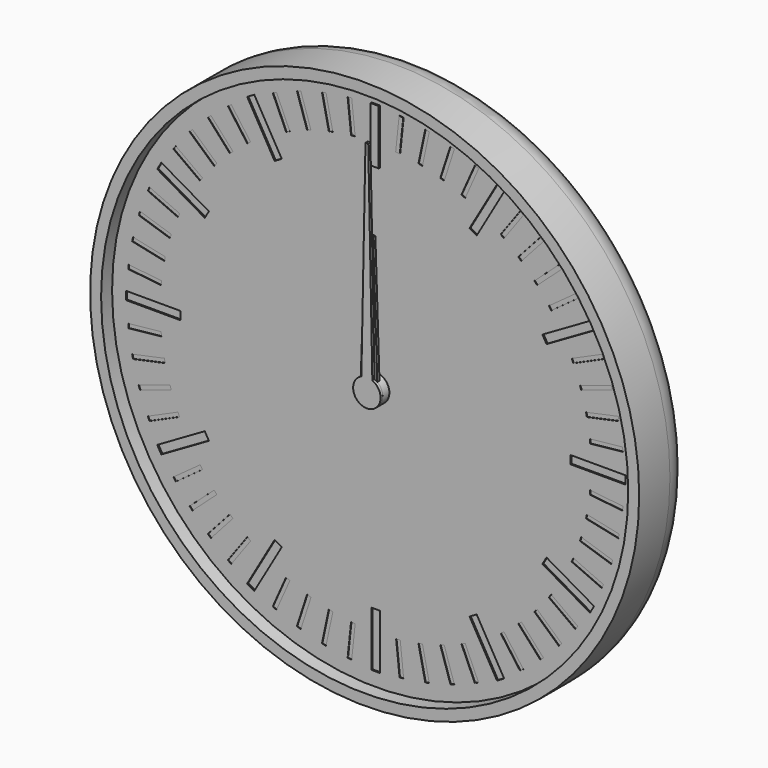
from build123d import *

# Parameters (mm, degrees)
F0_R      = 100
F1_DEPTH  = 24
F2_R      = 10
F3_T      = -4
F4_R      = 5
F4_R_2    = 3
F5_DEPTH  = 2
F6_DEPTH  = 19
F7_DEPTH  = 8
F9_DEPTH  = 4
F11_DEPTH = 4
F12_R     = 5
F12_R_2   = 3
F13_DEPTH = 2
F14_R     = 3
F15_DEPTH = 4
F17_DEPTH = 4
F18_R     = 3
F19_DEPTH = 2
F20_R     = 98
F20_R_2   = 5
F21_DEPTH = 1
F23_R     = 5
F23_R_2   = 3
F24_DEPTH = 2
F25_W     = 3
F25_H     = 20
F25_W_2   = 20
F25_H_2   = 3
F26_DEPTH = 0.5
F27_W     = 1.5
F27_H     = 12
F27_W_2   = 12
F27_H_2   = 1.5
F28_DEPTH = 0.2
F29_DEPTH = 1
F30_DEPTH = 0.4
F31_R     = 5
F31_R_2   = 3
F32_DEPTH = 5
F33_R     = 3
F34_DEPTH = 1
F36_DEPTH = 1


with BuildPart() as f1:
    # F0 (on Front) → F1 (new body)
    with BuildSketch(Plane.XZ):
        Circle(F0_R)
    extrude(amount=F1_DEPTH)

    # F2
    f2_edges = [f1.edges().sort_by_distance(p)[0] for p in [
        (-100, 0, 0),
    ]]
    fillet(f2_edges, radius=F2_R)

    # F3
    f3_openings = [f1.faces().sort_by_distance(p)[0] for p in [
        (0, -24, 0),
    ]]
    offset(amount=F3_T, openings=f3_openings)

    # F4 (on face) → F5 (join)
    with BuildSketch(Plane.XZ.offset(4)):
        Circle(F4_R)
        Circle(F4_R_2, mode=Mode.SUBTRACT)
        with Locations((40, 0)):
            Circle(F4_R)
        with Locations((40, 0)):
            Circle(F4_R_2, mode=Mode.SUBTRACT)
    extrude(amount=F5_DEPTH)


with BuildPart() as f6:
    # F6 (new): a face of the model
    f6_faces = [f1.part.faces().sort_by_distance(p)[0] for p in [
        (0, -4, 0),
    ]]
    extrude(f6_faces, amount=F6_DEPTH)

    # F8 (on face) → F9 (join)
    with BuildSketch(Plane.XZ.offset(6)):
        with BuildLine():
            ThreePointArc((9.2729637667, -1.3794085621), (9.3494561423, -0.6915886375), (9.375, 0))
            ThreePointArc((9.375, 0), (9.3494561423, 0.6915886375), (9.2729637667, 1.3794085621))
            ThreePointArc((9.2729637667, 1.3794085621), (8.9161548403, 2.8970343223), (8.3127812852, 4.3345463782))
            ThreePointArc((8.3127812852, 4.3345463782), (7.5845343223, 5.5104867402), (6.6911892658, 6.566476316))
            ThreePointArc((6.6911892658, 6.566476316), (5.5104867402, 7.5845343223), (4.1773988938, 8.3928519278))
            ThreePointArc((4.1773988938, 8.3928519278), (2.8970343223, 8.9161548403), (1.5536078905, 9.2453733036))
            ThreePointArc((1.5536078905, 9.2453733036), (0, 9.375), (-1.5536078905, 9.2453733036))
            ThreePointArc((-1.5536078905, 9.2453733036), (-2.8970343223, 8.9161548403), (-4.1773988938, 8.3928519278))
            ThreePointArc((-4.1773988938, 8.3928519278), (-5.5104867402, 7.5845343223), (-6.6911892658, 6.566476316))
            ThreePointArc((-6.6911892658, 6.566476316), (-7.5845343223, 5.5104867402), (-8.3127812852, 4.3345463782))
            ThreePointArc((-8.3127812852, 4.3345463782), (-8.9161548403, 2.8970343223), (-9.2729637667, 1.3794085621))
            ThreePointArc((-9.2729637667, 1.3794085621), (-9.375, 0), (-9.2729637667, -1.3794085621))
            ThreePointArc((-9.2729637667, -1.3794085621), (-8.9161548403, -2.8970343223), (-8.3127812852, -4.3345463782))
            ThreePointArc((-8.3127812852, -4.3345463782), (-7.5845343223, -5.5104867402), (-6.6911892658, -6.566476316))
            ThreePointArc((-6.6911892658, -6.566476316), (-5.5104867402, -7.5845343223), (-4.1773988938, -8.3928519278))
            ThreePointArc((-4.1773988938, -8.3928519278), (-2.8970343223, -8.9161548403), (-1.5536078905, -9.2453733036))
            ThreePointArc((-1.5536078905, -9.2453733036), (0, -9.375), (1.5536078905, -9.2453733036))
            ThreePointArc((1.5536078905, -9.2453733036), (2.8970343223, -8.9161548403), (4.1773988938, -8.3928519278))
            ThreePointArc((4.1773988938, -8.3928519278), (5.5104867402, -7.5845343223), (6.6911892658, -6.566476316))
            ThreePointArc((6.6911892658, -6.566476316), (7.5845343223, -5.5104867402), (8.3127812852, -4.3345463782))
            ThreePointArc((8.3127812852, -4.3345463782), (8.9161548403, -2.8970343223), (9.2729637667, -1.3794085621))
        make_face()
        with BuildLine():
            ThreePointArc((8.3127812852, 4.3345463782), (8.9161548403, 2.8970343223), (9.2729637667, 1.3794085621))
            Line((9.2729637667, 1.3794085621), (11.1823199426, 2.3946312492))
            Line((11.1823199426, 2.3946312492), (10.8182678729, 3.515068311))
            Line((10.8182678729, 3.515068311), (10.4542158031, 4.6355053728))
            Line((10.4542158031, 4.6355053728), (8.3127812852, 4.3345463782))
        make_face()
        with BuildLine():
            Line((11.1823199426, -2.3946312492), (9.2729637667, -1.3794085621))
            ThreePointArc((9.2729637667, -1.3794085621), (8.9161548403, -2.8970343223), (8.3127812852, -4.3345463782))
            Line((8.3127812852, -4.3345463782), (10.4542158031, -4.6355053728))
            Line((10.4542158031, -4.6355053728), (10.8182678729, -3.515068311))
            Line((10.8182678729, -3.515068311), (11.1823199426, -2.3946312492))
        make_face()
        with BuildLine():
            ThreePointArc((4.1773988938, 8.3928519278), (5.5104867402, 7.5845343223), (6.6911892658, 6.566476316))
            Line((6.6911892658, 6.566476316), (7.6391579371, 8.5101001246))
            Line((7.6391579371, 8.5101001246), (6.6860572448, 9.202568311))
            Line((6.6860572448, 9.202568311), (5.7329565525, 9.8950364974))
            Line((5.7329565525, 9.8950364974), (4.1773988938, 8.3928519278))
        make_face()
        with BuildLine():
            Line((7.6391579371, -8.5101001246), (6.6911892658, -6.566476316))
            ThreePointArc((6.6911892658, -6.566476316), (5.5104867402, -7.5845343223), (4.1773988938, -8.3928519278))
            Line((4.1773988938, -8.3928519278), (5.7329565525, -9.8950364974))
            Line((5.7329565525, -9.8950364974), (6.6860572448, -9.202568311))
            Line((6.6860572448, -9.202568311), (7.6391579371, -8.5101001246))
        make_face()
        with BuildLine():
            ThreePointArc((-1.5536078905, 9.2453733036), (0, 9.375), (1.5536078905, 9.2453733036))
            Line((1.5536078905, 9.2453733036), (1.1780972451, 11.375))
            Line((1.1780972451, 11.375), (0, 11.375))
            Line((0, 11.375), (-1.1780972451, 11.375))
            Line((-1.1780972451, 11.375), (-1.5536078905, 9.2453733036))
        make_face()
        with BuildLine():
            Line((1.1780972451, -11.375), (1.5536078905, -9.2453733036))
            ThreePointArc((1.5536078905, -9.2453733036), (0, -9.375), (-1.5536078905, -9.2453733036))
            Line((-1.5536078905, -9.2453733036), (-1.1780972451, -11.375))
            Line((-1.1780972451, -11.375), (0, -11.375))
            Line((0, -11.375), (1.1780972451, -11.375))
        make_face()
        with BuildLine():
            ThreePointArc((-6.6911892658, 6.566476316), (-5.5104867402, 7.5845343223), (-4.1773988938, 8.3928519278))
            Line((-4.1773988938, 8.3928519278), (-5.7329565525, 9.8950364974))
            Line((-5.7329565525, 9.8950364974), (-6.6860572448, 9.202568311))
            Line((-6.6860572448, 9.202568311), (-7.6391579371, 8.5101001246))
            Line((-7.6391579371, 8.5101001246), (-6.6911892658, 6.566476316))
        make_face()
        with BuildLine():
            Line((-5.7329565525, -9.8950364974), (-4.1773988938, -8.3928519278))
            ThreePointArc((-4.1773988938, -8.3928519278), (-5.5104867402, -7.5845343223), (-6.6911892658, -6.566476316))
            Line((-6.6911892658, -6.566476316), (-7.6391579371, -8.5101001246))
            Line((-7.6391579371, -8.5101001246), (-6.6860572448, -9.202568311))
            Line((-6.6860572448, -9.202568311), (-5.7329565525, -9.8950364974))
        make_face()
        with BuildLine():
            ThreePointArc((-9.2729637667, 1.3794085621), (-8.9161548403, 2.8970343223), (-8.3127812852, 4.3345463782))
            Line((-8.3127812852, 4.3345463782), (-10.4542158031, 4.6355053728))
            Line((-10.4542158031, 4.6355053728), (-10.8182678729, 3.515068311))
            Line((-10.8182678729, 3.515068311), (-11.1823199426, 2.3946312492))
            Line((-11.1823199426, 2.3946312492), (-9.2729637667, 1.3794085621))
        make_face()
        with BuildLine():
            Line((-10.4542158031, -4.6355053728), (-8.3127812852, -4.3345463782))
            ThreePointArc((-8.3127812852, -4.3345463782), (-8.9161548403, -2.8970343223), (-9.2729637667, -1.3794085621))
            Line((-9.2729637667, -1.3794085621), (-11.1823199426, -2.3946312492))
            Line((-11.1823199426, -2.3946312492), (-10.8182678729, -3.515068311))
            Line((-10.8182678729, -3.515068311), (-10.4542158031, -4.6355053728))
        make_face()
    extrude(amount=F9_DEPTH)

    # F35 (on face) → F36 (join)
    with BuildSketch(Plane.XZ.offset(23)):
        with BuildLine():
            ThreePointArc((-2, 4.582575695), (-2.7386127875, -4.1833001327), (5, 0))
            ThreePointArc((5, 0), (4.1833001327, 2.7386127875), (2, 4.582575695))
            ThreePointArc((2, 4.582575695), (0, 5), (-2, 4.582575695))
        make_face()
        with BuildLine():
            ThreePointArc((-2, 4.582575695), (0, 5), (2, 4.582575695))
            Line((2, 4.582575695), (0.5, 80))
            Line((0.5, 80), (0, 80))
            Line((0, 80), (-0.5, 80))
            Line((-0.5, 80), (-2, 4.582575695))
        make_face()
    extrude(amount=-F36_DEPTH)


with BuildPart() as f7:
    # F7 (new): a face of the model
    f7_faces = [f1.part.faces().sort_by_distance(p)[0] for p in [
        (40, -4, 0),
    ]]
    extrude(f7_faces, amount=F7_DEPTH)

    # F10 (on face) → F11 (join)
    with BuildSketch(Plane.XZ.offset(6)):
        with BuildLine():
            ThreePointArc((68.0829066802, -1.5381733945), (68.1144747006, -0.7693746225), (68.125, 0))
            ThreePointArc((68.125, 0), (68.1144747006, 0.7693746225), (68.0829066802, 1.5381733945))
            ThreePointArc((68.0829066802, 1.5381733945), (67.9709283072, 2.9398630294), (67.7890320221, 4.3342039956))
            ThreePointArc((67.7890320221, 4.3342039956), (67.5104012706, 5.8475163042), (67.1494235596, 7.3433252263))
            ThreePointArc((67.1494235596, 7.3433252263), (66.7484645208, 8.6911029668), (66.280643318, 10.0171558733))
            ThreePointArc((66.280643318, 10.0171558733), (65.6934659962, 11.4394680865), (65.0293803521, 12.8275385085))
            ThreePointArc((65.0293803521, 12.8275385085), (64.3569644814, 14.0625), (63.6236643925, 15.2623099717))
            ThreePointArc((63.6236643925, 15.2623099717), (62.7536029668, 16.5314602207), (61.815433119, 17.7511268046))
            ThreePointArc((61.815433119, 17.7511268046), (60.9009482166, 18.8192983038), (59.934217974, 19.8404278876))
            ThreePointArc((59.934217974, 19.8404278876), (58.8192983038, 20.9009482166), (57.6480467764, 21.8989056799))
            ThreePointArc((57.6480467764, 21.8989056799), (56.5314602207, 22.7536029668), (55.3735505752, 23.5514238999))
            ThreePointArc((55.3735505752, 23.5514238999), (54.0625, 24.3569644814), (52.709356105, 25.0895972944))
            ThreePointArc((52.709356105, 25.0895972944), (51.4394680865, 25.6934659962), (50.1409852457, 26.2331096755))
            ThreePointArc((50.1409852457, 26.2331096755), (48.6911029668, 26.7484645208), (47.2152055856, 27.1837531139))
            ThreePointArc((47.2152055856, 27.1837531139), (45.8475163042, 27.5104012706), (44.4652101991, 27.7682826779))
            ThreePointArc((44.4652101991, 27.7682826779), (42.9398630294, 27.9709283072), (41.4057159597, 28.0898484802))
            ThreePointArc((41.4057159597, 28.0898484802), (40, 28.125), (38.5942840403, 28.0898484802))
            ThreePointArc((38.5942840403, 28.0898484802), (37.0601369706, 27.9709283072), (35.5347898009, 27.7682826779))
            ThreePointArc((35.5347898009, 27.7682826779), (34.1524836958, 27.5104012706), (32.7847944144, 27.1837531139))
            ThreePointArc((32.7847944144, 27.1837531139), (31.3088970332, 26.7484645208), (29.8590147543, 26.2331096755))
            ThreePointArc((29.8590147543, 26.2331096755), (28.5605319135, 25.6934659962), (27.290643895, 25.0895972944))
            ThreePointArc((27.290643895, 25.0895972944), (25.9375, 24.3569644814), (24.6264494248, 23.5514238999))
            ThreePointArc((24.6264494248, 23.5514238999), (23.4685397793, 22.7536029668), (22.3519532236, 21.8989056799))
            ThreePointArc((22.3519532236, 21.8989056799), (21.1807016962, 20.9009482166), (20.065782026, 19.8404278876))
            ThreePointArc((20.065782026, 19.8404278876), (19.0990517834, 18.8192983038), (18.184566881, 17.7511268046))
            ThreePointArc((18.184566881, 17.7511268046), (17.2463970332, 16.5314602207), (16.3763356075, 15.2623099717))
            ThreePointArc((16.3763356075, 15.2623099717), (15.6430355186, 14.0625), (14.9706196479, 12.8275385085))
            ThreePointArc((14.9706196479, 12.8275385085), (14.3065340038, 11.4394680865), (13.719356682, 10.0171558733))
            ThreePointArc((13.719356682, 10.0171558733), (13.2515354792, 8.6911029668), (12.8505764404, 7.3433252263))
            ThreePointArc((12.8505764404, 7.3433252263), (12.4895987294, 5.8475163042), (12.2109679779, 4.3342039956))
            ThreePointArc((12.2109679779, 4.3342039956), (12.0290716928, 2.9398630294), (11.9170933198, 1.5381733945))
            ThreePointArc((11.9170933198, 1.5381733945), (11.875, 0), (11.9170933198, -1.5381733945))
            ThreePointArc((11.9170933198, -1.5381733945), (12.0290716928, -2.9398630294), (12.2109679779, -4.3342039956))
            ThreePointArc((12.2109679779, -4.3342039956), (12.4895987294, -5.8475163042), (12.8505764404, -7.3433252263))
            ThreePointArc((12.8505764404, -7.3433252263), (13.2515354792, -8.6911029668), (13.719356682, -10.0171558733))
            ThreePointArc((13.719356682, -10.0171558733), (14.3065340038, -11.4394680865), (14.9706196479, -12.8275385085))
            ThreePointArc((14.9706196479, -12.8275385085), (15.6430355186, -14.0625), (16.3763356075, -15.2623099717))
            ThreePointArc((16.3763356075, -15.2623099717), (17.2463970332, -16.5314602207), (18.184566881, -17.7511268046))
            ThreePointArc((18.184566881, -17.7511268046), (19.0990517834, -18.8192983038), (20.065782026, -19.8404278876))
            ThreePointArc((20.065782026, -19.8404278876), (21.1807016962, -20.9009482166), (22.3519532236, -21.8989056799))
            ThreePointArc((22.3519532236, -21.8989056799), (23.4685397793, -22.7536029668), (24.6264494248, -23.5514238999))
            ThreePointArc((24.6264494248, -23.5514238999), (25.9375, -24.3569644814), (27.290643895, -25.0895972944))
            ThreePointArc((27.290643895, -25.0895972944), (28.5605319135, -25.6934659962), (29.8590147543, -26.2331096755))
            ThreePointArc((29.8590147543, -26.2331096755), (31.3088970332, -26.7484645208), (32.7847944144, -27.1837531139))
            ThreePointArc((32.7847944144, -27.1837531139), (34.1524836958, -27.5104012706), (35.5347898009, -27.7682826779))
            ThreePointArc((35.5347898009, -27.7682826779), (37.0601369706, -27.9709283072), (38.5942840403, -28.0898484802))
            ThreePointArc((38.5942840403, -28.0898484802), (40, -28.125), (41.4057159597, -28.0898484802))
            ThreePointArc((41.4057159597, -28.0898484802), (42.9398630294, -27.9709283072), (44.4652101991, -27.7682826779))
            ThreePointArc((44.4652101991, -27.7682826779), (45.8475163042, -27.5104012706), (47.2152055856, -27.1837531139))
            ThreePointArc((47.2152055856, -27.1837531139), (48.6911029668, -26.7484645208), (50.1409852457, -26.2331096755))
            ThreePointArc((50.1409852457, -26.2331096755), (51.4394680865, -25.6934659962), (52.709356105, -25.0895972944))
            ThreePointArc((52.709356105, -25.0895972944), (54.0625, -24.3569644814), (55.3735505752, -23.5514238999))
            ThreePointArc((55.3735505752, -23.5514238999), (56.5314602207, -22.7536029668), (57.6480467764, -21.8989056799))
            ThreePointArc((57.6480467764, -21.8989056799), (58.8192983038, -20.9009482166), (59.934217974, -19.8404278876))
            ThreePointArc((59.934217974, -19.8404278876), (60.9009482166, -18.8192983038), (61.815433119, -17.7511268046))
            ThreePointArc((61.815433119, -17.7511268046), (62.7536029668, -16.5314602207), (63.6236643925, -15.2623099717))
            ThreePointArc((63.6236643925, -15.2623099717), (64.3569644814, -14.0625), (65.0293803521, -12.8275385085))
            ThreePointArc((65.0293803521, -12.8275385085), (65.6934659962, -11.4394680865), (66.280643318, -10.0171558733))
            ThreePointArc((66.280643318, -10.0171558733), (66.7484645208, -8.6911029668), (67.1494235596, -7.3433252263))
            ThreePointArc((67.1494235596, -7.3433252263), (67.5104012706, -5.8475163042), (67.7890320221, -4.3342039956))
            ThreePointArc((67.7890320221, -4.3342039956), (67.9709283072, -2.9398630294), (68.0829066802, -1.5381733945))
        make_face()
        with BuildLine():
            ThreePointArc((68.0829066802, 1.5381733945), (68.1144747006, 0.7693746225), (68.125, 0))
            ThreePointArc((68.125, 0), (68.1144747006, -0.7693746225), (68.0829066802, -1.5381733945))
            Line((68.0829066802, -1.5381733945), (70.125, -1.1780972451))
            Line((70.125, -1.1780972451), (70.125, 0))
            Line((70.125, 0), (70.125, 1.1780972451))
            Line((70.125, 1.1780972451), (68.0829066802, 1.5381733945))
        make_face()
        with BuildLine():
            ThreePointArc((67.1494235596, 7.3433252263), (67.5104012706, 5.8475163042), (67.7890320221, 4.3342039956))
            Line((67.7890320221, 4.3342039956), (69.7116366623, 5.1109866922))
            Line((69.7116366623, 5.1109866922), (69.4666964721, 6.2633396859))
            Line((69.4666964721, 6.2633396859), (69.2217562819, 7.4156926796))
            Line((69.2217562819, 7.4156926796), (67.1494235596, 7.3433252263))
        make_face()
        with BuildLine():
            Line((69.7116366623, -5.1109866922), (67.7890320221, -4.3342039956))
            ThreePointArc((67.7890320221, -4.3342039956), (67.5104012706, -5.8475163042), (67.1494235596, -7.3433252263))
            Line((67.1494235596, -7.3433252263), (69.2217562819, -7.4156926796))
            Line((69.2217562819, -7.4156926796), (69.4666964721, -6.2633396859))
            Line((69.4666964721, -6.2633396859), (69.7116366623, -5.1109866922))
        make_face()
        with BuildLine():
            ThreePointArc((65.0293803521, 12.8275385085), (65.6934659962, 11.4394680865), (66.280643318, 10.0171558733))
            Line((66.280643318, 10.0171558733), (67.9997322302, 11.1766959857))
            Line((67.9997322302, 11.1766959857), (67.5205569115, 12.2529413727))
            Line((67.5205569115, 12.2529413727), (67.0413815928, 13.3291867596))
            Line((67.0413815928, 13.3291867596), (65.0293803521, 12.8275385085))
        make_face()
        with BuildLine():
            Line((67.9997322302, -11.1766959857), (66.280643318, -10.0171558733))
            ThreePointArc((66.280643318, -10.0171558733), (65.6934659962, -11.4394680865), (65.0293803521, -12.8275385085))
            Line((65.0293803521, -12.8275385085), (67.0413815928, -13.3291867596))
            Line((67.0413815928, -13.3291867596), (67.5205569115, -12.2529413727))
            Line((67.5205569115, -12.2529413727), (67.9997322302, -11.1766959857))
        make_face()
        with BuildLine():
            ThreePointArc((61.815433119, 17.7511268046), (62.7536029668, 16.5314602207), (63.6236643925, 15.2623099717))
            Line((63.6236643925, 15.2623099717), (65.064105142, 16.753930033))
            Line((65.064105142, 16.753930033), (64.3716369555, 17.7070307253))
            Line((64.3716369555, 17.7070307253), (63.6791687691, 18.6601314176))
            Line((63.6791687691, 18.6601314176), (61.815433119, 17.7511268046))
        make_face()
        with BuildLine():
            Line((65.064105142, -16.753930033), (63.6236643925, -15.2623099717))
            ThreePointArc((63.6236643925, -15.2623099717), (62.7536029668, -16.5314602207), (61.815433119, -17.7511268046))
            Line((61.815433119, -17.7511268046), (63.6791687691, -18.6601314176))
            Line((63.6791687691, -18.6601314176), (64.3716369555, -17.7070307253))
            Line((64.3716369555, -17.7070307253), (65.064105142, -16.753930033))
        make_face()
        with BuildLine():
            ThreePointArc((57.6480467764, 21.8989056799), (58.8192983038, 20.9009482166), (59.934217974, 19.8404278876))
            Line((59.934217974, 19.8404278876), (61.0330563882, 21.5989369435))
            Line((61.0330563882, 21.5989369435), (60.1575595166, 22.3872378675))
            Line((60.1575595166, 22.3872378675), (59.282062645, 23.1755387915))
            Line((59.282062645, 23.1755387915), (57.6480467764, 21.8989056799))
        make_face()
        with BuildLine():
            Line((61.0330563882, -21.5989369435), (59.934217974, -19.8404278876))
            ThreePointArc((59.934217974, -19.8404278876), (58.8192983038, -20.9009482166), (57.6480467764, -21.8989056799))
            Line((57.6480467764, -21.8989056799), (59.282062645, -23.1755387915))
            Line((59.282062645, -23.1755387915), (60.1575595166, -22.3872378675))
            Line((60.1575595166, -22.3872378675), (61.0330563882, -21.5989369435))
        make_face()
        with BuildLine():
            ThreePointArc((52.709356105, 25.0895972944), (54.0625, 24.3569644814), (55.3735505752, 23.5514238999))
            Line((55.3735505752, 23.5514238999), (56.0827621424, 25.4999666665))
            Line((56.0827621424, 25.4999666665), (55.0625, 26.089015289))
            Line((55.0625, 26.089015289), (54.0422378576, 26.6780639116))
            Line((54.0422378576, 26.6780639116), (52.709356105, 25.0895972944))
        make_face()
        with BuildLine():
            Line((56.0827621424, -25.4999666665), (55.3735505752, -23.5514238999))
            ThreePointArc((55.3735505752, -23.5514238999), (54.0625, -24.3569644814), (52.709356105, -25.0895972944))
            Line((52.709356105, -25.0895972944), (54.0422378576, -26.6780639116))
            Line((54.0422378576, -26.6780639116), (55.0625, -26.089015289))
            Line((55.0625, -26.089015289), (56.0827621424, -25.4999666665))
        make_face()
        with BuildLine():
            ThreePointArc((47.2152055856, 27.1837531139), (48.6911029668, 26.7484645208), (50.1409852457, 26.2331096755))
            Line((50.1409852457, 26.2331096755), (50.4295740173, 28.2865254836))
            Line((50.4295740173, 28.2865254836), (49.3091369555, 28.6505775534))
            Line((49.3091369555, 28.6505775534), (48.1886998938, 29.0146296232))
            Line((48.1886998938, 29.0146296232), (47.2152055856, 27.1837531139))
        make_face()
        with BuildLine():
            Line((50.4295740173, -28.2865254836), (50.1409852457, -26.2331096755))
            ThreePointArc((50.1409852457, -26.2331096755), (48.6911029668, -26.7484645208), (47.2152055856, -27.1837531139))
            Line((47.2152055856, -27.1837531139), (48.1886998938, -29.0146296232))
            Line((48.1886998938, -29.0146296232), (49.3091369555, -28.6505775534))
            Line((49.3091369555, -28.6505775534), (50.4295740173, -28.2865254836))
        make_face()
        with BuildLine():
            ThreePointArc((41.4057159597, 28.0898484802), (42.9398630294, 27.9709283072), (44.4652101991, 27.7682826779))
            Line((44.4652101991, 27.7682826779), (44.3205634611, 29.8368274034))
            Line((44.3205634611, 29.8368274034), (43.1489199559, 29.959972098))
            Line((43.1489199559, 29.959972098), (41.9772764508, 30.0831167926))
            Line((41.9772764508, 30.0831167926), (41.4057159597, 28.0898484802))
        make_face()
        with BuildLine():
            Line((44.3205634611, -29.8368274034), (44.4652101991, -27.7682826779))
            ThreePointArc((44.4652101991, -27.7682826779), (42.9398630294, -27.9709283072), (41.4057159597, -28.0898484802))
            Line((41.4057159597, -28.0898484802), (41.9772764508, -30.0831167926))
            Line((41.9772764508, -30.0831167926), (43.1489199559, -29.959972098))
            Line((43.1489199559, -29.959972098), (44.3205634611, -29.8368274034))
        make_face()
        with BuildLine():
            ThreePointArc((35.5347898009, 27.7682826779), (37.0601369706, 27.9709283072), (38.5942840403, 28.0898484802))
            Line((38.5942840403, 28.0898484802), (38.0227235492, 30.0831167926))
            Line((38.0227235492, 30.0831167926), (36.8510800441, 29.959972098))
            Line((36.8510800441, 29.959972098), (35.6794365389, 29.8368274034))
            Line((35.6794365389, 29.8368274034), (35.5347898009, 27.7682826779))
        make_face()
        with BuildLine():
            Line((38.0227235492, -30.0831167926), (38.5942840403, -28.0898484802))
            ThreePointArc((38.5942840403, -28.0898484802), (37.0601369706, -27.9709283072), (35.5347898009, -27.7682826779))
            Line((35.5347898009, -27.7682826779), (35.6794365389, -29.8368274034))
            Line((35.6794365389, -29.8368274034), (36.8510800441, -29.959972098))
            Line((36.8510800441, -29.959972098), (38.0227235492, -30.0831167926))
        make_face()
        with BuildLine():
            ThreePointArc((29.8590147543, 26.2331096755), (31.3088970332, 26.7484645208), (32.7847944144, 27.1837531139))
            Line((32.7847944144, 27.1837531139), (31.8113001062, 29.0146296232))
            Line((31.8113001062, 29.0146296232), (30.6908630445, 28.6505775534))
            Line((30.6908630445, 28.6505775534), (29.5704259827, 28.2865254836))
            Line((29.5704259827, 28.2865254836), (29.8590147543, 26.2331096755))
        make_face()
        with BuildLine():
            Line((31.8113001062, -29.0146296232), (32.7847944144, -27.1837531139))
            ThreePointArc((32.7847944144, -27.1837531139), (31.3088970332, -26.7484645208), (29.8590147543, -26.2331096755))
            Line((29.8590147543, -26.2331096755), (29.5704259827, -28.2865254836))
            Line((29.5704259827, -28.2865254836), (30.6908630445, -28.6505775534))
            Line((30.6908630445, -28.6505775534), (31.8113001062, -29.0146296232))
        make_face()
        with BuildLine():
            ThreePointArc((24.6264494248, 23.5514238999), (25.9375, 24.3569644814), (27.290643895, 25.0895972944))
            Line((27.290643895, 25.0895972944), (25.9577621424, 26.6780639116))
            Line((25.9577621424, 26.6780639116), (24.9375, 26.089015289))
            Line((24.9375, 26.089015289), (23.9172378576, 25.4999666665))
            Line((23.9172378576, 25.4999666665), (24.6264494248, 23.5514238999))
        make_face()
        with BuildLine():
            Line((25.9577621424, -26.6780639116), (27.290643895, -25.0895972944))
            ThreePointArc((27.290643895, -25.0895972944), (25.9375, -24.3569644814), (24.6264494248, -23.5514238999))
            Line((24.6264494248, -23.5514238999), (23.9172378576, -25.4999666665))
            Line((23.9172378576, -25.4999666665), (24.9375, -26.089015289))
            Line((24.9375, -26.089015289), (25.9577621424, -26.6780639116))
        make_face()
        with BuildLine():
            ThreePointArc((20.065782026, 19.8404278876), (21.1807016962, 20.9009482166), (22.3519532236, 21.8989056799))
            Line((22.3519532236, 21.8989056799), (20.717937355, 23.1755387915))
            Line((20.717937355, 23.1755387915), (19.8424404834, 22.3872378675))
            Line((19.8424404834, 22.3872378675), (18.9669436118, 21.5989369435))
            Line((18.9669436118, 21.5989369435), (20.065782026, 19.8404278876))
        make_face()
        with BuildLine():
            Line((20.717937355, -23.1755387915), (22.3519532236, -21.8989056799))
            ThreePointArc((22.3519532236, -21.8989056799), (21.1807016962, -20.9009482166), (20.065782026, -19.8404278876))
            Line((20.065782026, -19.8404278876), (18.9669436118, -21.5989369435))
            Line((18.9669436118, -21.5989369435), (19.8424404834, -22.3872378675))
            Line((19.8424404834, -22.3872378675), (20.717937355, -23.1755387915))
        make_face()
        with BuildLine():
            ThreePointArc((16.3763356075, 15.2623099717), (17.2463970332, 16.5314602207), (18.184566881, 17.7511268046))
            Line((18.184566881, 17.7511268046), (16.3208312309, 18.6601314176))
            Line((16.3208312309, 18.6601314176), (15.6283630445, 17.7070307253))
            Line((15.6283630445, 17.7070307253), (14.935894858, 16.753930033))
            Line((14.935894858, 16.753930033), (16.3763356075, 15.2623099717))
        make_face()
        with BuildLine():
            Line((16.3208312309, -18.6601314176), (18.184566881, -17.7511268046))
            ThreePointArc((18.184566881, -17.7511268046), (17.2463970332, -16.5314602207), (16.3763356075, -15.2623099717))
            Line((16.3763356075, -15.2623099717), (14.935894858, -16.753930033))
            Line((14.935894858, -16.753930033), (15.6283630445, -17.7070307253))
            Line((15.6283630445, -17.7070307253), (16.3208312309, -18.6601314176))
        make_face()
        with BuildLine():
            ThreePointArc((13.719356682, 10.0171558733), (14.3065340038, 11.4394680865), (14.9706196479, 12.8275385085))
            Line((14.9706196479, 12.8275385085), (12.9586184072, 13.3291867596))
            Line((12.9586184072, 13.3291867596), (12.4794430885, 12.2529413727))
            Line((12.4794430885, 12.2529413727), (12.0002677698, 11.1766959857))
            Line((12.0002677698, 11.1766959857), (13.719356682, 10.0171558733))
        make_face()
        with BuildLine():
            Line((12.9586184072, -13.3291867596), (14.9706196479, -12.8275385085))
            ThreePointArc((14.9706196479, -12.8275385085), (14.3065340038, -11.4394680865), (13.719356682, -10.0171558733))
            Line((13.719356682, -10.0171558733), (12.0002677698, -11.1766959857))
            Line((12.0002677698, -11.1766959857), (12.4794430885, -12.2529413727))
            Line((12.4794430885, -12.2529413727), (12.9586184072, -13.3291867596))
        make_face()
        with BuildLine():
            ThreePointArc((12.2109679779, 4.3342039956), (12.4895987294, 5.8475163042), (12.8505764404, 7.3433252263))
            Line((12.8505764404, 7.3433252263), (10.7782437181, 7.4156926796))
            Line((10.7782437181, 7.4156926796), (10.5333035279, 6.2633396859))
            Line((10.5333035279, 6.2633396859), (10.2883633377, 5.1109866922))
            Line((10.2883633377, 5.1109866922), (12.2109679779, 4.3342039956))
        make_face()
        with BuildLine():
            Line((10.7782437181, -7.4156926796), (12.8505764404, -7.3433252263))
            ThreePointArc((12.8505764404, -7.3433252263), (12.4895987294, -5.8475163042), (12.2109679779, -4.3342039956))
            Line((12.2109679779, -4.3342039956), (10.2883633377, -5.1109866922))
            Line((10.2883633377, -5.1109866922), (10.5333035279, -6.2633396859))
            Line((10.5333035279, -6.2633396859), (10.7782437181, -7.4156926796))
        make_face()
        with BuildLine():
            ThreePointArc((11.9170933198, -1.5381733945), (11.875, 0), (11.9170933198, 1.5381733945))
            Line((11.9170933198, 1.5381733945), (9.875, 1.1780972451))
            Line((9.875, 1.1780972451), (9.875, 0))
            Line((9.875, 0), (9.875, -1.1780972451))
            Line((9.875, -1.1780972451), (11.9170933198, -1.5381733945))
        make_face()
    extrude(amount=F11_DEPTH)

    # F16 (on face) → F17 (join)
    with BuildSketch(Plane.XZ.offset(12)):
        with BuildLine():
            ThreePointArc((47.4288750323, -1.0304444454), (47.4821976298, -0.5164480894), (47.5, 0))
            ThreePointArc((47.5, 0), (47.4821976298, 0.5164480894), (47.4288750323, 1.0304444454))
            ThreePointArc((47.4288750323, 1.0304444454), (47.1329238722, 2.3176274578), (46.6157661985, 3.532936117))
            ThreePointArc((46.6157661985, 3.532936117), (46.0676274578, 4.4083893922), (45.4044061018, 5.2002302532))
            ThreePointArc((45.4044061018, 5.2002302532), (44.4083893922, 6.0676274578), (43.2756595386, 6.7468551628))
            ThreePointArc((43.2756595386, 6.7468551628), (42.3176274578, 7.1329238722), (41.3156377295, 7.3837048536))
            ThreePointArc((41.3156377295, 7.3837048536), (40, 7.5), (38.6843622705, 7.3837048536))
            ThreePointArc((38.6843622705, 7.3837048536), (37.6823725422, 7.1329238722), (36.7243404614, 6.7468551628))
            ThreePointArc((36.7243404614, 6.7468551628), (35.5916106078, 6.0676274578), (34.5955938982, 5.2002302532))
            ThreePointArc((34.5955938982, 5.2002302532), (33.9323725422, 4.4083893922), (33.3842338015, 3.532936117))
            ThreePointArc((33.3842338015, 3.532936117), (32.8670761278, 2.3176274578), (32.5711249677, 1.0304444454))
            ThreePointArc((32.5711249677, 1.0304444454), (32.5, 0), (32.5711249677, -1.0304444454))
            ThreePointArc((32.5711249677, -1.0304444454), (32.8670761278, -2.3176274578), (33.3842338015, -3.532936117))
            ThreePointArc((33.3842338015, -3.532936117), (33.9323725422, -4.4083893922), (34.5955938982, -5.2002302532))
            ThreePointArc((34.5955938982, -5.2002302532), (35.5916106078, -6.0676274578), (36.7243404614, -6.7468551628))
            ThreePointArc((36.7243404614, -6.7468551628), (37.6823725422, -7.1329238722), (38.6843622705, -7.3837048536))
            ThreePointArc((38.6843622705, -7.3837048536), (40, -7.5), (41.3156377295, -7.3837048536))
            ThreePointArc((41.3156377295, -7.3837048536), (42.3176274578, -7.1329238722), (43.2756595386, -6.7468551628))
            ThreePointArc((43.2756595386, -6.7468551628), (44.4083893922, -6.0676274578), (45.4044061018, -5.2002302532))
            ThreePointArc((45.4044061018, -5.2002302532), (46.0676274578, -4.4083893922), (46.6157661985, -3.532936117))
            ThreePointArc((46.6157661985, -3.532936117), (47.1329238722, -2.3176274578), (47.4288750323, -1.0304444454))
        make_face()
        with BuildLine():
            ThreePointArc((46.6157661985, 3.532936117), (47.1329238722, 2.3176274578), (47.4288750323, 1.0304444454))
            Line((47.4288750323, 1.0304444454), (49.3262785606, 2.0393117971))
            Line((49.3262785606, 2.0393117971), (48.743795249, 3.832011096))
            Line((48.743795249, 3.832011096), (46.6157661985, 3.532936117))
        make_face()
        with BuildLine():
            Line((49.3262785606, -2.0393117971), (47.4288750323, -1.0304444454))
            ThreePointArc((47.4288750323, -1.0304444454), (47.1329238722, -2.3176274578), (46.6157661985, -3.532936117))
            Line((46.6157661985, -3.532936117), (48.743795249, -3.832011096))
            Line((48.743795249, -3.832011096), (49.3262785606, -2.0393117971))
        make_face()
        with BuildLine():
            ThreePointArc((43.2756595386, 6.7468551628), (44.4083893922, 6.0676274578), (45.4044061018, 5.2002302532))
            Line((45.4044061018, 5.2002302532), (46.3464404506, 7.1316868974))
            Line((46.3464404506, 7.1316868974), (44.8214793429, 8.2396359957))
            Line((44.8214793429, 8.2396359957), (43.2756595386, 6.7468551628))
        make_face()
        with BuildLine():
            Line((46.3464404506, -7.1316868974), (45.4044061018, -5.2002302532))
            ThreePointArc((45.4044061018, -5.2002302532), (44.4083893922, -6.0676274578), (43.2756595386, -6.7468551628))
            Line((43.2756595386, -6.7468551628), (44.8214793429, -8.2396359957))
            Line((44.8214793429, -8.2396359957), (46.3464404506, -7.1316868974))
        make_face()
        with BuildLine():
            ThreePointArc((38.6843622705, 7.3837048536), (40, 7.5), (41.3156377295, 7.3837048536))
            Line((41.3156377295, 7.3837048536), (40.9424777961, 9.5))
            Line((40.9424777961, 9.5), (39.0575222039, 9.5))
            Line((39.0575222039, 9.5), (38.6843622705, 7.3837048536))
        make_face()
        with BuildLine():
            Line((40.9424777961, -9.5), (41.3156377295, -7.3837048536))
            ThreePointArc((41.3156377295, -7.3837048536), (40, -7.5), (38.6843622705, -7.3837048536))
            Line((38.6843622705, -7.3837048536), (39.0575222039, -9.5))
            Line((39.0575222039, -9.5), (40.9424777961, -9.5))
        make_face()
        with BuildLine():
            ThreePointArc((34.5955938982, 5.2002302532), (35.5916106078, 6.0676274578), (36.7243404614, 6.7468551628))
            Line((36.7243404614, 6.7468551628), (35.1785206571, 8.2396359957))
            Line((35.1785206571, 8.2396359957), (33.6535595494, 7.1316868974))
            Line((33.6535595494, 7.1316868974), (34.5955938982, 5.2002302532))
        make_face()
        with BuildLine():
            Line((35.1785206571, -8.2396359957), (36.7243404614, -6.7468551628))
            ThreePointArc((36.7243404614, -6.7468551628), (35.5916106078, -6.0676274578), (34.5955938982, -5.2002302532))
            Line((34.5955938982, -5.2002302532), (33.6535595494, -7.1316868974))
            Line((33.6535595494, -7.1316868974), (35.1785206571, -8.2396359957))
        make_face()
        with BuildLine():
            ThreePointArc((32.5711249677, 1.0304444454), (32.8670761278, 2.3176274578), (33.3842338015, 3.532936117))
            Line((33.3842338015, 3.532936117), (31.256204751, 3.832011096))
            Line((31.256204751, 3.832011096), (30.6737214394, 2.0393117971))
            Line((30.6737214394, 2.0393117971), (32.5711249677, 1.0304444454))
        make_face()
        with BuildLine():
            Line((31.256204751, -3.832011096), (33.3842338015, -3.532936117))
            ThreePointArc((33.3842338015, -3.532936117), (32.8670761278, -2.3176274578), (32.5711249677, -1.0304444454))
            Line((32.5711249677, -1.0304444454), (30.6737214394, -2.0393117971))
            Line((30.6737214394, -2.0393117971), (31.256204751, -3.832011096))
        make_face()
    extrude(amount=F17_DEPTH)

    # F18 (on face) → F19 (join)
    with BuildSketch(Plane.XZ.offset(16)):
        with Locations((40, 0)):
            Circle(F18_R)
    extrude(amount=F19_DEPTH)


with BuildPart() as f13:
    # F12 (on face) → F13 (new body)
    with BuildSketch(Plane.XZ.offset(10)):
        Circle(F12_R)
        Circle(F12_R_2, mode=Mode.SUBTRACT)
    extrude(amount=F13_DEPTH)

    # F14 (on face) → F15 (join)
    with BuildSketch(Plane.XZ.offset(12)):
        with BuildLine():
            ThreePointArc((29.9718156995, -1.3001014101), (29.9929530972, -0.6502034357), (30, 0))
            ThreePointArc((30, 0), (29.9929530972, 0.6502034357), (29.9718156995, 1.3001014101))
            ThreePointArc((29.9718156995, 1.3001014101), (29.907520012, 2.3537728718), (29.8061935814, 3.4045299509))
            ThreePointArc((29.8061935814, 3.4045299509), (29.6306502179, 4.6930339512), (29.3994322443, 5.9727199596))
            ThreePointArc((29.3994322443, 5.9727199596), (29.1710976119, 7.0033609157), (28.9066440563, 8.0253304855))
            ThreePointArc((28.9066440563, 8.0253304855), (28.5316954889, 9.2705098312), (28.1031371961, 10.4982703213))
            ThreePointArc((28.1031371961, 10.4982703213), (27.7163859753, 11.480502971), (27.2953170189, 12.448520749))
            ThreePointArc((27.2953170189, 12.448520749), (26.7301957257, 13.6197149922), (26.1148496411, 14.765318426))
            ThreePointArc((26.1148496411, 14.765318426), (25.5792049306, 15.6749569415), (25.0118886885, 16.5651871174))
            ThreePointArc((25.0118886885, 16.5651871174), (24.2705098312, 17.6335575688), (23.4835278178, 18.6687953878))
            ThreePointArc((23.4835278178, 18.6687953878), (22.812178968, 19.4834414499), (22.1125846489, 20.2739636023))
            ThreePointArc((22.1125846489, 20.2739636023), (21.2132034356, 21.2132034356), (20.2739636023, 22.1125846489))
            ThreePointArc((20.2739636023, 22.1125846489), (19.4834414499, 22.812178968), (18.6687953878, 23.4835278178))
            ThreePointArc((18.6687953878, 23.4835278178), (17.6335575688, 24.2705098312), (16.5651871174, 25.0118886885))
            ThreePointArc((16.5651871174, 25.0118886885), (15.6749569415, 25.5792049306), (14.765318426, 26.1148496411))
            ThreePointArc((14.765318426, 26.1148496411), (13.6197149922, 26.7301957257), (12.448520749, 27.2953170189))
            ThreePointArc((12.448520749, 27.2953170189), (11.480502971, 27.7163859753), (10.4982703213, 28.1031371961))
            ThreePointArc((10.4982703213, 28.1031371961), (9.2705098312, 28.5316954889), (8.0253304855, 28.9066440563))
            ThreePointArc((8.0253304855, 28.9066440563), (7.0033609157, 29.1710976119), (5.9727199596, 29.3994322443))
            ThreePointArc((5.9727199596, 29.3994322443), (4.6930339512, 29.6306502179), (3.4045299509, 29.8061935814))
            ThreePointArc((3.4045299509, 29.8061935814), (2.3537728718, 29.907520012), (1.3001014101, 29.9718156995))
            ThreePointArc((1.3001014101, 29.9718156995), (0, 30), (-1.3001014101, 29.9718156995))
            ThreePointArc((-1.3001014101, 29.9718156995), (-2.3537728718, 29.907520012), (-3.4045299509, 29.8061935814))
            ThreePointArc((-3.4045299509, 29.8061935814), (-4.6930339512, 29.6306502179), (-5.9727199596, 29.3994322443))
            ThreePointArc((-5.9727199596, 29.3994322443), (-7.0033609157, 29.1710976119), (-8.0253304855, 28.9066440563))
            ThreePointArc((-8.0253304855, 28.9066440563), (-9.2705098312, 28.5316954889), (-10.4982703213, 28.1031371961))
            ThreePointArc((-10.4982703213, 28.1031371961), (-11.480502971, 27.7163859753), (-12.448520749, 27.2953170189))
            ThreePointArc((-12.448520749, 27.2953170189), (-13.6197149922, 26.7301957257), (-14.765318426, 26.1148496411))
            ThreePointArc((-14.765318426, 26.1148496411), (-15.6749569415, 25.5792049306), (-16.5651871174, 25.0118886885))
            ThreePointArc((-16.5651871174, 25.0118886885), (-17.6335575688, 24.2705098312), (-18.6687953878, 23.4835278178))
            ThreePointArc((-18.6687953878, 23.4835278178), (-19.4834414499, 22.812178968), (-20.2739636023, 22.1125846489))
            ThreePointArc((-20.2739636023, 22.1125846489), (-21.2132034356, 21.2132034356), (-22.1125846489, 20.2739636023))
            ThreePointArc((-22.1125846489, 20.2739636023), (-22.812178968, 19.4834414499), (-23.4835278178, 18.6687953878))
            ThreePointArc((-23.4835278178, 18.6687953878), (-24.2705098312, 17.6335575688), (-25.0118886885, 16.5651871174))
            ThreePointArc((-25.0118886885, 16.5651871174), (-25.5792049306, 15.6749569415), (-26.1148496411, 14.765318426))
            ThreePointArc((-26.1148496411, 14.765318426), (-26.7301957257, 13.6197149922), (-27.2953170189, 12.448520749))
            ThreePointArc((-27.2953170189, 12.448520749), (-27.7163859753, 11.480502971), (-28.1031371961, 10.4982703213))
            ThreePointArc((-28.1031371961, 10.4982703213), (-28.5316954889, 9.2705098312), (-28.9066440563, 8.0253304855))
            ThreePointArc((-28.9066440563, 8.0253304855), (-29.1710976119, 7.0033609157), (-29.3994322443, 5.9727199596))
            ThreePointArc((-29.3994322443, 5.9727199596), (-29.6306502179, 4.6930339512), (-29.8061935814, 3.4045299509))
            ThreePointArc((-29.8061935814, 3.4045299509), (-29.907520012, 2.3537728718), (-29.9718156995, 1.3001014101))
            ThreePointArc((-29.9718156995, 1.3001014101), (-30, 0), (-29.9718156995, -1.3001014101))
            ThreePointArc((-29.9718156995, -1.3001014101), (-29.907520012, -2.3537728718), (-29.8061935814, -3.4045299509))
            ThreePointArc((-29.8061935814, -3.4045299509), (-29.6306502179, -4.6930339512), (-29.3994322443, -5.9727199596))
            ThreePointArc((-29.3994322443, -5.9727199596), (-29.1710976119, -7.0033609157), (-28.9066440563, -8.0253304855))
            ThreePointArc((-28.9066440563, -8.0253304855), (-28.5316954889, -9.2705098312), (-28.1031371961, -10.4982703213))
            ThreePointArc((-28.1031371961, -10.4982703213), (-27.7163859753, -11.480502971), (-27.2953170189, -12.448520749))
            ThreePointArc((-27.2953170189, -12.448520749), (-26.7301957257, -13.6197149922), (-26.1148496411, -14.765318426))
            ThreePointArc((-26.1148496411, -14.765318426), (-25.5792049306, -15.6749569415), (-25.0118886885, -16.5651871174))
            ThreePointArc((-25.0118886885, -16.5651871174), (-24.2705098312, -17.6335575688), (-23.4835278178, -18.6687953878))
            ThreePointArc((-23.4835278178, -18.6687953878), (-22.812178968, -19.4834414499), (-22.1125846489, -20.2739636023))
            ThreePointArc((-22.1125846489, -20.2739636023), (-21.2132034356, -21.2132034356), (-20.2739636023, -22.1125846489))
            ThreePointArc((-20.2739636023, -22.1125846489), (-19.4834414499, -22.812178968), (-18.6687953878, -23.4835278178))
            ThreePointArc((-18.6687953878, -23.4835278178), (-17.6335575688, -24.2705098312), (-16.5651871174, -25.0118886885))
            ThreePointArc((-16.5651871174, -25.0118886885), (-15.6749569415, -25.5792049306), (-14.765318426, -26.1148496411))
            ThreePointArc((-14.765318426, -26.1148496411), (-13.6197149922, -26.7301957257), (-12.448520749, -27.2953170189))
            ThreePointArc((-12.448520749, -27.2953170189), (-11.480502971, -27.7163859753), (-10.4982703213, -28.1031371961))
            ThreePointArc((-10.4982703213, -28.1031371961), (-9.2705098312, -28.5316954889), (-8.0253304855, -28.9066440563))
            ThreePointArc((-8.0253304855, -28.9066440563), (-7.0033609157, -29.1710976119), (-5.9727199596, -29.3994322443))
            ThreePointArc((-5.9727199596, -29.3994322443), (-4.6930339512, -29.6306502179), (-3.4045299509, -29.8061935814))
            ThreePointArc((-3.4045299509, -29.8061935814), (-2.3537728718, -29.907520012), (-1.3001014101, -29.9718156995))
            ThreePointArc((-1.3001014101, -29.9718156995), (0, -30), (1.3001014101, -29.9718156995))
            ThreePointArc((1.3001014101, -29.9718156995), (2.3537728718, -29.907520012), (3.4045299509, -29.8061935814))
            ThreePointArc((3.4045299509, -29.8061935814), (4.6930339512, -29.6306502179), (5.9727199596, -29.3994322443))
            ThreePointArc((5.9727199596, -29.3994322443), (7.0033609157, -29.1710976119), (8.0253304855, -28.9066440563))
            ThreePointArc((8.0253304855, -28.9066440563), (9.2705098312, -28.5316954889), (10.4982703213, -28.1031371961))
            ThreePointArc((10.4982703213, -28.1031371961), (11.480502971, -27.7163859753), (12.448520749, -27.2953170189))
            ThreePointArc((12.448520749, -27.2953170189), (13.6197149922, -26.7301957257), (14.765318426, -26.1148496411))
            ThreePointArc((14.765318426, -26.1148496411), (15.6749569415, -25.5792049306), (16.5651871174, -25.0118886885))
            ThreePointArc((16.5651871174, -25.0118886885), (17.6335575688, -24.2705098312), (18.6687953878, -23.4835278178))
            ThreePointArc((18.6687953878, -23.4835278178), (19.4834414499, -22.812178968), (20.2739636023, -22.1125846489))
            ThreePointArc((20.2739636023, -22.1125846489), (21.2132034356, -21.2132034356), (22.1125846489, -20.2739636023))
            ThreePointArc((22.1125846489, -20.2739636023), (22.812178968, -19.4834414499), (23.4835278178, -18.6687953878))
            ThreePointArc((23.4835278178, -18.6687953878), (24.2705098312, -17.6335575688), (25.0118886885, -16.5651871174))
            ThreePointArc((25.0118886885, -16.5651871174), (25.5792049306, -15.6749569415), (26.1148496411, -14.765318426))
            ThreePointArc((26.1148496411, -14.765318426), (26.7301957257, -13.6197149922), (27.2953170189, -12.448520749))
            ThreePointArc((27.2953170189, -12.448520749), (27.7163859753, -11.480502971), (28.1031371961, -10.4982703213))
            ThreePointArc((28.1031371961, -10.4982703213), (28.5316954889, -9.2705098312), (28.9066440563, -8.0253304855))
            ThreePointArc((28.9066440563, -8.0253304855), (29.1710976119, -7.0033609157), (29.3994322443, -5.9727199596))
            ThreePointArc((29.3994322443, -5.9727199596), (29.6306502179, -4.6930339512), (29.8061935814, -3.4045299509))
            ThreePointArc((29.8061935814, -3.4045299509), (29.907520012, -2.3537728718), (29.9718156995, -1.3001014101))
        make_face()
        Circle(F14_R, mode=Mode.SUBTRACT)
        with BuildLine():
            ThreePointArc((29.9718156995, 1.3001014101), (29.9929530972, 0.6502034357), (30, 0))
            ThreePointArc((30, 0), (29.9929530972, -0.6502034357), (29.9718156995, -1.3001014101))
            Line((29.9718156995, -1.3001014101), (32, -0.9424777961))
            Line((32, -0.9424777961), (32, 0))
            Line((32, 0), (32, 0.9424777961))
            Line((32, 0.9424777961), (29.9718156995, 1.3001014101))
        make_face()
        with BuildLine():
            ThreePointArc((29.3994322443, 5.9727199596), (29.6306502179, 4.6930339512), (29.8061935814, 3.4045299509))
            Line((29.8061935814, 3.4045299509), (31.7534629089, 4.0750285508))
            Line((31.7534629089, 4.0750285508), (31.606026899, 5.0059028813))
            Line((31.606026899, 5.0059028813), (31.4585908892, 5.9367772117))
            Line((31.4585908892, 5.9367772117), (29.3994322443, 5.9727199596))
        make_face()
        with BuildLine():
            Line((31.7534629089, -4.0750285508), (29.8061935814, -3.4045299509))
            ThreePointArc((29.8061935814, -3.4045299509), (29.6306502179, -4.6930339512), (29.3994322443, -5.9727199596))
            Line((29.3994322443, -5.9727199596), (31.4585908892, -5.9367772117))
            Line((31.4585908892, -5.9367772117), (31.606026899, -5.0059028813))
            Line((31.606026899, -5.0059028813), (31.7534629089, -4.0750285508))
        make_face()
        with BuildLine():
            ThreePointArc((28.1031371961, 10.4982703213), (28.5316954889, 9.2705098312), (28.9066440563, 8.0253304855))
            Line((28.9066440563, 8.0253304855), (30.7250501773, 8.9921941706))
            Line((30.7250501773, 8.9921941706), (30.4338085214, 9.88854382))
            Line((30.4338085214, 9.88854382), (30.1425668656, 10.7848934694))
            Line((30.1425668656, 10.7848934694), (28.1031371961, 10.4982703213))
        make_face()
        with BuildLine():
            Line((30.7250501773, -8.9921941706), (28.9066440563, -8.0253304855))
            ThreePointArc((28.9066440563, -8.0253304855), (28.5316954889, -9.2705098312), (28.1031371961, -10.4982703213))
            Line((28.1031371961, -10.4982703213), (30.1425668656, -10.7848934694))
            Line((30.1425668656, -10.7848934694), (30.4338085214, -9.88854382))
            Line((30.4338085214, -9.88854382), (30.7250501773, -8.9921941706))
        make_face()
        with BuildLine():
            ThreePointArc((26.1148496411, 14.765318426), (26.7301957257, 13.6197149922), (27.2953170189, 12.448520749))
            Line((27.2953170189, 12.448520749), (28.9400847397, 13.6879421265))
            Line((28.9400847397, 13.6879421265), (28.512208774, 14.5276959917))
            Line((28.512208774, 14.5276959917), (28.0843328084, 15.3674498569))
            Line((28.0843328084, 15.3674498569), (26.1148496411, 14.765318426))
        make_face()
        with BuildLine():
            Line((28.9400847397, -13.6879421265), (27.2953170189, -12.448520749))
            ThreePointArc((27.2953170189, -12.448520749), (26.7301957257, -13.6197149922), (26.1148496411, -14.765318426))
            Line((26.1148496411, -14.765318426), (28.0843328084, -15.3674498569))
            Line((28.0843328084, -15.3674498569), (28.512208774, -14.5276959917))
            Line((28.512208774, -14.5276959917), (28.9400847397, -13.6879421265))
        make_face()
        with BuildLine():
            ThreePointArc((23.4835278178, 18.6687953878), (24.2705098312, 17.6335575688), (25.0118886885, 16.5651871174))
            Line((25.0118886885, 16.5651871174), (26.4425183691, 18.0466475195))
            Line((26.4425183691, 18.0466475195), (25.88854382, 18.8091280734))
            Line((25.88854382, 18.8091280734), (25.3345692709, 19.5716086272))
            Line((25.3345692709, 19.5716086272), (23.4835278178, 18.6687953878))
        make_face()
        with BuildLine():
            Line((26.4425183691, -18.0466475195), (25.0118886885, -16.5651871174))
            ThreePointArc((25.0118886885, -16.5651871174), (24.2705098312, -17.6335575688), (23.4835278178, -18.6687953878))
            Line((23.4835278178, -18.6687953878), (25.3345692709, -19.5716086272))
            Line((25.3345692709, -19.5716086272), (25.88854382, -18.8091280734))
            Line((25.88854382, -18.8091280734), (26.4425183691, -18.0466475195))
        make_face()
        with BuildLine():
            ThreePointArc((20.2739636023, 22.1125846489), (21.2132034356, 21.2132034356), (22.1125846489, 20.2739636023))
            Line((22.1125846489, 20.2739636023), (23.2938494387, 21.9609845572))
            Line((23.2938494387, 21.9609845572), (22.627416998, 22.627416998))
            Line((22.627416998, 22.627416998), (21.9609845572, 23.2938494387))
            Line((21.9609845572, 23.2938494387), (20.2739636023, 22.1125846489))
        make_face()
        with BuildLine():
            Line((23.2938494387, -21.9609845572), (22.1125846489, -20.2739636023))
            ThreePointArc((22.1125846489, -20.2739636023), (21.2132034356, -21.2132034356), (20.2739636023, -22.1125846489))
            Line((20.2739636023, -22.1125846489), (21.9609845572, -23.2938494387))
            Line((21.9609845572, -23.2938494387), (22.627416998, -22.627416998))
            Line((22.627416998, -22.627416998), (23.2938494387, -21.9609845572))
        make_face()
        with BuildLine():
            ThreePointArc((16.5651871174, 25.0118886885), (17.6335575688, 24.2705098312), (18.6687953878, 23.4835278178))
            Line((18.6687953878, 23.4835278178), (19.5716086272, 25.3345692709))
            Line((19.5716086272, 25.3345692709), (18.8091280734, 25.88854382))
            Line((18.8091280734, 25.88854382), (18.0466475195, 26.4425183691))
            Line((18.0466475195, 26.4425183691), (16.5651871174, 25.0118886885))
        make_face()
        with BuildLine():
            Line((19.5716086272, -25.3345692709), (18.6687953878, -23.4835278178))
            ThreePointArc((18.6687953878, -23.4835278178), (17.6335575688, -24.2705098312), (16.5651871174, -25.0118886885))
            Line((16.5651871174, -25.0118886885), (18.0466475195, -26.4425183691))
            Line((18.0466475195, -26.4425183691), (18.8091280734, -25.88854382))
            Line((18.8091280734, -25.88854382), (19.5716086272, -25.3345692709))
        make_face()
        with BuildLine():
            ThreePointArc((12.448520749, 27.2953170189), (13.6197149922, 26.7301957257), (14.765318426, 26.1148496411))
            Line((14.765318426, 26.1148496411), (15.3674498569, 28.0843328084))
            Line((15.3674498569, 28.0843328084), (14.5276959917, 28.512208774))
            Line((14.5276959917, 28.512208774), (13.6879421265, 28.9400847397))
            Line((13.6879421265, 28.9400847397), (12.448520749, 27.2953170189))
        make_face()
        with BuildLine():
            Line((15.3674498569, -28.0843328084), (14.765318426, -26.1148496411))
            ThreePointArc((14.765318426, -26.1148496411), (13.6197149922, -26.7301957257), (12.448520749, -27.2953170189))
            Line((12.448520749, -27.2953170189), (13.6879421265, -28.9400847397))
            Line((13.6879421265, -28.9400847397), (14.5276959917, -28.512208774))
            Line((14.5276959917, -28.512208774), (15.3674498569, -28.0843328084))
        make_face()
        with BuildLine():
            ThreePointArc((8.0253304855, 28.9066440563), (9.2705098312, 28.5316954889), (10.4982703213, 28.1031371961))
            Line((10.4982703213, 28.1031371961), (10.7848934694, 30.1425668656))
            Line((10.7848934694, 30.1425668656), (9.88854382, 30.4338085214))
            Line((9.88854382, 30.4338085214), (8.9921941706, 30.7250501773))
            Line((8.9921941706, 30.7250501773), (8.0253304855, 28.9066440563))
        make_face()
        with BuildLine():
            Line((10.7848934694, -30.1425668656), (10.4982703213, -28.1031371961))
            ThreePointArc((10.4982703213, -28.1031371961), (9.2705098312, -28.5316954889), (8.0253304855, -28.9066440563))
            Line((8.0253304855, -28.9066440563), (8.9921941706, -30.7250501773))
            Line((8.9921941706, -30.7250501773), (9.88854382, -30.4338085214))
            Line((9.88854382, -30.4338085214), (10.7848934694, -30.1425668656))
        make_face()
        with BuildLine():
            ThreePointArc((3.4045299509, 29.8061935814), (4.6930339512, 29.6306502179), (5.9727199596, 29.3994322443))
            Line((5.9727199596, 29.3994322443), (5.9367772117, 31.4585908892))
            Line((5.9367772117, 31.4585908892), (5.0059028813, 31.606026899))
            Line((5.0059028813, 31.606026899), (4.0750285508, 31.7534629089))
            Line((4.0750285508, 31.7534629089), (3.4045299509, 29.8061935814))
        make_face()
        with BuildLine():
            Line((5.9367772117, -31.4585908892), (5.9727199596, -29.3994322443))
            ThreePointArc((5.9727199596, -29.3994322443), (4.6930339512, -29.6306502179), (3.4045299509, -29.8061935814))
            Line((3.4045299509, -29.8061935814), (4.0750285508, -31.7534629089))
            Line((4.0750285508, -31.7534629089), (5.0059028813, -31.606026899))
            Line((5.0059028813, -31.606026899), (5.9367772117, -31.4585908892))
        make_face()
        with BuildLine():
            ThreePointArc((-1.3001014101, 29.9718156995), (0, 30), (1.3001014101, 29.9718156995))
            Line((1.3001014101, 29.9718156995), (0.9424777961, 32))
            Line((0.9424777961, 32), (0, 32))
            Line((0, 32), (-0.9424777961, 32))
            Line((-0.9424777961, 32), (-1.3001014101, 29.9718156995))
        make_face()
        with BuildLine():
            Line((0.9424777961, -32), (1.3001014101, -29.9718156995))
            ThreePointArc((1.3001014101, -29.9718156995), (0, -30), (-1.3001014101, -29.9718156995))
            Line((-1.3001014101, -29.9718156995), (-0.9424777961, -32))
            Line((-0.9424777961, -32), (0, -32))
            Line((0, -32), (0.9424777961, -32))
        make_face()
        with BuildLine():
            ThreePointArc((-5.9727199596, 29.3994322443), (-4.6930339512, 29.6306502179), (-3.4045299509, 29.8061935814))
            Line((-3.4045299509, 29.8061935814), (-4.0750285508, 31.7534629089))
            Line((-4.0750285508, 31.7534629089), (-5.0059028813, 31.606026899))
            Line((-5.0059028813, 31.606026899), (-5.9367772117, 31.4585908892))
            Line((-5.9367772117, 31.4585908892), (-5.9727199596, 29.3994322443))
        make_face()
        with BuildLine():
            Line((-4.0750285508, -31.7534629089), (-3.4045299509, -29.8061935814))
            ThreePointArc((-3.4045299509, -29.8061935814), (-4.6930339512, -29.6306502179), (-5.9727199596, -29.3994322443))
            Line((-5.9727199596, -29.3994322443), (-5.9367772117, -31.4585908892))
            Line((-5.9367772117, -31.4585908892), (-5.0059028813, -31.606026899))
            Line((-5.0059028813, -31.606026899), (-4.0750285508, -31.7534629089))
        make_face()
        with BuildLine():
            ThreePointArc((-10.4982703213, 28.1031371961), (-9.2705098312, 28.5316954889), (-8.0253304855, 28.9066440563))
            Line((-8.0253304855, 28.9066440563), (-8.9921941706, 30.7250501773))
            Line((-8.9921941706, 30.7250501773), (-9.88854382, 30.4338085214))
            Line((-9.88854382, 30.4338085214), (-10.7848934694, 30.1425668656))
            Line((-10.7848934694, 30.1425668656), (-10.4982703213, 28.1031371961))
        make_face()
        with BuildLine():
            Line((-8.9921941706, -30.7250501773), (-8.0253304855, -28.9066440563))
            ThreePointArc((-8.0253304855, -28.9066440563), (-9.2705098312, -28.5316954889), (-10.4982703213, -28.1031371961))
            Line((-10.4982703213, -28.1031371961), (-10.7848934694, -30.1425668656))
            Line((-10.7848934694, -30.1425668656), (-9.88854382, -30.4338085214))
            Line((-9.88854382, -30.4338085214), (-8.9921941706, -30.7250501773))
        make_face()
        with BuildLine():
            ThreePointArc((-14.765318426, 26.1148496411), (-13.6197149922, 26.7301957257), (-12.448520749, 27.2953170189))
            Line((-12.448520749, 27.2953170189), (-13.6879421265, 28.9400847397))
            Line((-13.6879421265, 28.9400847397), (-14.5276959917, 28.512208774))
            Line((-14.5276959917, 28.512208774), (-15.3674498569, 28.0843328084))
            Line((-15.3674498569, 28.0843328084), (-14.765318426, 26.1148496411))
        make_face()
        with BuildLine():
            Line((-13.6879421265, -28.9400847397), (-12.448520749, -27.2953170189))
            ThreePointArc((-12.448520749, -27.2953170189), (-13.6197149922, -26.7301957257), (-14.765318426, -26.1148496411))
            Line((-14.765318426, -26.1148496411), (-15.3674498569, -28.0843328084))
            Line((-15.3674498569, -28.0843328084), (-14.5276959917, -28.512208774))
            Line((-14.5276959917, -28.512208774), (-13.6879421265, -28.9400847397))
        make_face()
        with BuildLine():
            ThreePointArc((-18.6687953878, 23.4835278178), (-17.6335575688, 24.2705098312), (-16.5651871174, 25.0118886885))
            Line((-16.5651871174, 25.0118886885), (-18.0466475195, 26.4425183691))
            Line((-18.0466475195, 26.4425183691), (-18.8091280734, 25.88854382))
            Line((-18.8091280734, 25.88854382), (-19.5716086272, 25.3345692709))
            Line((-19.5716086272, 25.3345692709), (-18.6687953878, 23.4835278178))
        make_face()
        with BuildLine():
            Line((-18.0466475195, -26.4425183691), (-16.5651871174, -25.0118886885))
            ThreePointArc((-16.5651871174, -25.0118886885), (-17.6335575688, -24.2705098312), (-18.6687953878, -23.4835278178))
            Line((-18.6687953878, -23.4835278178), (-19.5716086272, -25.3345692709))
            Line((-19.5716086272, -25.3345692709), (-18.8091280734, -25.88854382))
            Line((-18.8091280734, -25.88854382), (-18.0466475195, -26.4425183691))
        make_face()
        with BuildLine():
            ThreePointArc((-22.1125846489, 20.2739636023), (-21.2132034356, 21.2132034356), (-20.2739636023, 22.1125846489))
            Line((-20.2739636023, 22.1125846489), (-21.9609845572, 23.2938494387))
            Line((-21.9609845572, 23.2938494387), (-22.627416998, 22.627416998))
            Line((-22.627416998, 22.627416998), (-23.2938494387, 21.9609845572))
            Line((-23.2938494387, 21.9609845572), (-22.1125846489, 20.2739636023))
        make_face()
        with BuildLine():
            Line((-21.9609845572, -23.2938494387), (-20.2739636023, -22.1125846489))
            ThreePointArc((-20.2739636023, -22.1125846489), (-21.2132034356, -21.2132034356), (-22.1125846489, -20.2739636023))
            Line((-22.1125846489, -20.2739636023), (-23.2938494387, -21.9609845572))
            Line((-23.2938494387, -21.9609845572), (-22.627416998, -22.627416998))
            Line((-22.627416998, -22.627416998), (-21.9609845572, -23.2938494387))
        make_face()
        with BuildLine():
            ThreePointArc((-25.0118886885, 16.5651871174), (-24.2705098312, 17.6335575688), (-23.4835278178, 18.6687953878))
            Line((-23.4835278178, 18.6687953878), (-25.3345692709, 19.5716086272))
            Line((-25.3345692709, 19.5716086272), (-25.88854382, 18.8091280734))
            Line((-25.88854382, 18.8091280734), (-26.4425183691, 18.0466475195))
            Line((-26.4425183691, 18.0466475195), (-25.0118886885, 16.5651871174))
        make_face()
        with BuildLine():
            Line((-25.3345692709, -19.5716086272), (-23.4835278178, -18.6687953878))
            ThreePointArc((-23.4835278178, -18.6687953878), (-24.2705098312, -17.6335575688), (-25.0118886885, -16.5651871174))
            Line((-25.0118886885, -16.5651871174), (-26.4425183691, -18.0466475195))
            Line((-26.4425183691, -18.0466475195), (-25.88854382, -18.8091280734))
            Line((-25.88854382, -18.8091280734), (-25.3345692709, -19.5716086272))
        make_face()
        with BuildLine():
            ThreePointArc((-27.2953170189, 12.448520749), (-26.7301957257, 13.6197149922), (-26.1148496411, 14.765318426))
            Line((-26.1148496411, 14.765318426), (-28.0843328084, 15.3674498569))
            Line((-28.0843328084, 15.3674498569), (-28.512208774, 14.5276959917))
            Line((-28.512208774, 14.5276959917), (-28.9400847397, 13.6879421265))
            Line((-28.9400847397, 13.6879421265), (-27.2953170189, 12.448520749))
        make_face()
        with BuildLine():
            Line((-28.0843328084, -15.3674498569), (-26.1148496411, -14.765318426))
            ThreePointArc((-26.1148496411, -14.765318426), (-26.7301957257, -13.6197149922), (-27.2953170189, -12.448520749))
            Line((-27.2953170189, -12.448520749), (-28.9400847397, -13.6879421265))
            Line((-28.9400847397, -13.6879421265), (-28.512208774, -14.5276959917))
            Line((-28.512208774, -14.5276959917), (-28.0843328084, -15.3674498569))
        make_face()
        with BuildLine():
            ThreePointArc((-28.9066440563, 8.0253304855), (-28.5316954889, 9.2705098312), (-28.1031371961, 10.4982703213))
            Line((-28.1031371961, 10.4982703213), (-30.1425668656, 10.7848934694))
            Line((-30.1425668656, 10.7848934694), (-30.4338085214, 9.88854382))
            Line((-30.4338085214, 9.88854382), (-30.7250501773, 8.9921941706))
            Line((-30.7250501773, 8.9921941706), (-28.9066440563, 8.0253304855))
        make_face()
        with BuildLine():
            Line((-30.1425668656, -10.7848934694), (-28.1031371961, -10.4982703213))
            ThreePointArc((-28.1031371961, -10.4982703213), (-28.5316954889, -9.2705098312), (-28.9066440563, -8.0253304855))
            Line((-28.9066440563, -8.0253304855), (-30.7250501773, -8.9921941706))
            Line((-30.7250501773, -8.9921941706), (-30.4338085214, -9.88854382))
            Line((-30.4338085214, -9.88854382), (-30.1425668656, -10.7848934694))
        make_face()
        with BuildLine():
            ThreePointArc((-29.8061935814, 3.4045299509), (-29.6306502179, 4.6930339512), (-29.3994322443, 5.9727199596))
            Line((-29.3994322443, 5.9727199596), (-31.4585908892, 5.9367772117))
            Line((-31.4585908892, 5.9367772117), (-31.606026899, 5.0059028813))
            Line((-31.606026899, 5.0059028813), (-31.7534629089, 4.0750285508))
            Line((-31.7534629089, 4.0750285508), (-29.8061935814, 3.4045299509))
        make_face()
        with BuildLine():
            Line((-31.4585908892, -5.9367772117), (-29.3994322443, -5.9727199596))
            ThreePointArc((-29.3994322443, -5.9727199596), (-29.6306502179, -4.6930339512), (-29.8061935814, -3.4045299509))
            Line((-29.8061935814, -3.4045299509), (-31.7534629089, -4.0750285508))
            Line((-31.7534629089, -4.0750285508), (-31.606026899, -5.0059028813))
            Line((-31.606026899, -5.0059028813), (-31.4585908892, -5.9367772117))
        make_face()
        with BuildLine():
            ThreePointArc((-29.9718156995, -1.3001014101), (-30, 0), (-29.9718156995, 1.3001014101))
            Line((-29.9718156995, 1.3001014101), (-32, 0.9424777961))
            Line((-32, 0.9424777961), (-32, 0))
            Line((-32, 0), (-32, -0.9424777961))
            Line((-32, -0.9424777961), (-29.9718156995, -1.3001014101))
        make_face()
    extrude(amount=F15_DEPTH)

    # F31 (on face) → F32 (join)
    with BuildSketch(Plane.XZ.offset(16)):
        Circle(F31_R)
        Circle(F31_R_2, mode=Mode.SUBTRACT)
    extrude(amount=F32_DEPTH)

    # F33 (on face) → F34 (join)
    with BuildSketch(Plane.XZ.offset(21)):
        with BuildLine():
            ThreePointArc((-3, 4), (-2.2360679775, -4.472135955), (5, 0))
            ThreePointArc((5, 0), (4.472135955, 2.2360679775), (3, 4))
            ThreePointArc((3, 4), (0, 5), (-3, 4))
        make_face()
        Circle(F33_R, mode=Mode.SUBTRACT)
        with BuildLine():
            ThreePointArc((-3, 4), (0, 5), (3, 4))
            Line((3, 4), (1.5, 50))
            Line((1.5, 50), (0, 50))
            Line((0, 50), (-1.5, 50))
            Line((-1.5, 50), (-3, 4))
        make_face()
    extrude(amount=F34_DEPTH)


with BuildPart() as f21:
    # F20 (on face) → F21 (new body)
    with BuildSketch(Plane.XZ.offset(18)):
        Circle(F20_R)
        Circle(F20_R_2, mode=Mode.SUBTRACT)
    extrude(amount=F21_DEPTH)


with BuildPart() as f1_1:
    add(f1.part)

    # F22: cut F21
    add(f21.part, mode=Mode.SUBTRACT)


with BuildPart() as f21_1:
    add(f21.part)

    # F23 (on face) → F24 (join, through all)
    with BuildSketch(Plane(origin=(0, -18, 0), x_dir=(-1, 0, 0), z_dir=(0, 1, 0))):
        with Locations((-40, 0)):
            Circle(F23_R)
        with Locations((-40, 0)):
            Circle(F23_R_2, mode=Mode.SUBTRACT)
    extrude(amount=F24_DEPTH)

    # F25 (on face) → F26 (cut)
    with BuildSketch(Plane.XZ.offset(19)):
        with Locations((0, 81)):
            Rectangle(F25_W, F25_H)
        Polygon((-46.7990381057, 78.0583117444), (-36.7990381057, 60.7378036687), (-34.2009618943, 62.2378036687), (-44.2009618943, 79.5583117444), align=None)
        Polygon((-79.5583117444, 44.2009618943), (-62.2378036687, 34.2009618943), (-60.7378036687, 36.7990381057), (-78.0583117444, 46.7990381057), align=None)
        with Locations((-81, 0)):
            Rectangle(F25_W_2, F25_H_2)
        Polygon((-78.0583117444, -46.7990381057), (-60.7378036687, -36.7990381057), (-62.2378036687, -34.2009618943), (-79.5583117444, -44.2009618943), align=None)
        Polygon((-44.2009618943, -79.5583117444), (-34.2009618943, -62.2378036687), (-36.7990381057, -60.7378036687), (-46.7990381057, -78.0583117444), align=None)
        with Locations((0, -81)):
            Rectangle(F25_W, F25_H)
        Polygon((46.7990381057, -78.0583117444), (36.7990381057, -60.7378036687), (34.2009618943, -62.2378036687), (44.2009618943, -79.5583117444), align=None)
        Polygon((79.5583117444, -44.2009618943), (62.2378036687, -34.2009618943), (60.7378036687, -36.7990381057), (78.0583117444, -46.7990381057), align=None)
        with Locations((81, 0)):
            Rectangle(F25_W_2, F25_H_2)
        Polygon((78.0583117444, 46.7990381057), (60.7378036687, 36.7990381057), (62.2378036687, 34.2009618943), (79.5583117444, 44.2009618943), align=None)
        Polygon((44.2009618943, 79.5583117444), (34.2009618943, 62.2378036687), (36.7990381057, 60.7378036687), (46.7990381057, 78.0583117444), align=None)
    extrude(amount=-F26_DEPTH, mode=Mode.SUBTRACT)

    # F27 (on face) → F28 (cut)
    with BuildSketch(Plane.XZ.offset(19)):
        with Locations((0, 84.5)):
            Rectangle(F27_W, F27_H)
        Polygon((-7.459592945, 78.1483651339), (-8.7139345042, 90.0826278783), (-10.2057173472, 89.9258351834), (-8.951375788, 77.991572439), align=None)
        Polygon((-15.5874570286, 76.9405204257), (-18.0823973185, 88.6782916345), (-19.5496187196, 88.3664240983), (-17.0546784297, 76.6286528895), align=None)
        Polygon((-23.5445416712, 74.889699275), (-27.2527456037, 86.3023774705), (-28.6793303782, 85.8388519789), (-24.9711264457, 74.4261737834), align=None)
        Polygon((-31.2436673882, 72.0183709073), (-36.1245071051, 82.980916399), (-37.4948252916, 82.3708114343), (-32.6139855747, 71.4082659426), align=None)
        Polygon((-38.6004809472, 68.3579941971), (-44.6004809472, 78.7502990425), (-45.8995190528, 78.0002990425), (-39.8995190528, 67.6079941971), align=None)
        Polygon((-45.5343795592, 63.9486729977), (-52.5878025867, 73.6568769302), (-53.8013280783, 72.7751990517), (-46.7479050507, 63.0669951192), align=None)
        Polygon((-51.9693939801, 58.8387167547), (-59.9989612564, 67.7564546605), (-61.1136784946, 66.7527587509), (-53.0841112183, 57.8350208452), align=None)
        Polygon((-57.8350208452, 53.0841112183), (-66.7527587509, 61.1136784946), (-67.7564546605, 59.9989612564), (-58.8387167547, 51.9693939801), align=None)
        Polygon((-63.0669951192, 46.7479050507), (-72.7751990517, 53.8013280783), (-73.6568769302, 52.5878025867), (-63.9486729977, 45.5343795592), align=None)
        Polygon((-67.6079941971, 39.8995190528), (-78.0002990425, 45.8995190528), (-78.7502990425, 44.6004809472), (-68.3579941971, 38.6004809472), align=None)
        Polygon((-71.4082659426, 32.6139855747), (-82.3708114343, 37.4948252916), (-82.980916399, 36.1245071051), (-72.0183709073, 31.2436673882), align=None)
        Polygon((-74.4261737834, 24.9711264457), (-85.8388519789, 28.6793303782), (-86.3023774705, 27.2527456037), (-74.889699275, 23.5445416712), align=None)
        Polygon((-76.6286528895, 17.0546784297), (-88.3664240983, 19.5496187196), (-88.6782916345, 18.0823973185), (-76.9405204257, 15.5874570286), align=None)
        Polygon((-77.991572439, 8.951375788), (-89.9258351834, 10.2057173472), (-90.0826278783, 8.7139345042), (-78.1483651339, 7.459592945), align=None)
        with Locations((-84.5, 0)):
            Rectangle(F27_W_2, F27_H_2)
        Polygon((-78.1483651339, -7.459592945), (-90.0826278783, -8.7139345042), (-89.9258351834, -10.2057173472), (-77.991572439, -8.951375788), align=None)
        Polygon((-76.9405204257, -15.5874570286), (-88.6782916345, -18.0823973185), (-88.3664240983, -19.5496187196), (-76.6286528895, -17.0546784297), align=None)
        Polygon((-74.889699275, -23.5445416712), (-86.3023774705, -27.2527456037), (-85.8388519789, -28.6793303782), (-74.4261737834, -24.9711264457), align=None)
        Polygon((-72.0183709073, -31.2436673882), (-82.980916399, -36.1245071051), (-82.3708114343, -37.4948252916), (-71.4082659426, -32.6139855747), align=None)
        Polygon((-68.3579941971, -38.6004809472), (-78.7502990425, -44.6004809472), (-78.0002990425, -45.8995190528), (-67.6079941971, -39.8995190528), align=None)
        Polygon((-63.9486729977, -45.5343795592), (-73.6568769302, -52.5878025867), (-72.7751990517, -53.8013280783), (-63.0669951192, -46.7479050507), align=None)
        Polygon((-58.8387167547, -51.9693939801), (-67.7564546605, -59.9989612564), (-66.7527587509, -61.1136784946), (-57.8350208452, -53.0841112183), align=None)
        Polygon((-53.0841112183, -57.8350208452), (-61.1136784946, -66.7527587509), (-59.9989612564, -67.7564546605), (-51.9693939801, -58.8387167547), align=None)
        Polygon((-46.7479050507, -63.0669951192), (-53.8013280783, -72.7751990517), (-52.5878025867, -73.6568769302), (-45.5343795592, -63.9486729977), align=None)
        Polygon((-39.8995190528, -67.6079941971), (-45.8995190528, -78.0002990425), (-44.6004809472, -78.7502990425), (-38.6004809472, -68.3579941971), align=None)
        Polygon((-32.6139855747, -71.4082659426), (-37.4948252916, -82.3708114343), (-36.1245071051, -82.980916399), (-31.2436673882, -72.0183709073), align=None)
        Polygon((-24.9711264457, -74.4261737834), (-28.6793303782, -85.8388519789), (-27.2527456037, -86.3023774705), (-23.5445416712, -74.889699275), align=None)
        Polygon((-17.0546784297, -76.6286528895), (-19.5496187196, -88.3664240983), (-18.0823973185, -88.6782916345), (-15.5874570286, -76.9405204257), align=None)
        Polygon((-8.951375788, -77.991572439), (-10.2057173472, -89.9258351834), (-8.7139345042, -90.0826278783), (-7.459592945, -78.1483651339), align=None)
        with Locations((0, -84.5)):
            Rectangle(F27_W, F27_H)
        Polygon((7.459592945, -78.1483651339), (8.7139345042, -90.0826278783), (10.2057173472, -89.9258351834), (8.951375788, -77.991572439), align=None)
        Polygon((15.5874570286, -76.9405204257), (18.0823973185, -88.6782916345), (19.5496187196, -88.3664240983), (17.0546784297, -76.6286528895), align=None)
        Polygon((23.5445416712, -74.889699275), (27.2527456037, -86.3023774705), (28.6793303782, -85.8388519789), (24.9711264457, -74.4261737834), align=None)
        Polygon((31.2436673882, -72.0183709073), (36.1245071051, -82.980916399), (37.4948252916, -82.3708114343), (32.6139855747, -71.4082659426), align=None)
        Polygon((38.6004809472, -68.3579941971), (44.6004809472, -78.7502990425), (45.8995190528, -78.0002990425), (39.8995190528, -67.6079941971), align=None)
        Polygon((45.5343795592, -63.9486729977), (52.5878025867, -73.6568769302), (53.8013280783, -72.7751990517), (46.7479050507, -63.0669951192), align=None)
        Polygon((51.9693939801, -58.8387167547), (59.9989612564, -67.7564546605), (61.1136784946, -66.7527587509), (53.0841112183, -57.8350208452), align=None)
        Polygon((57.8350208452, -53.0841112183), (66.7527587509, -61.1136784946), (67.7564546605, -59.9989612564), (58.8387167547, -51.9693939801), align=None)
        Polygon((63.0669951192, -46.7479050507), (72.7751990517, -53.8013280783), (73.6568769302, -52.5878025867), (63.9486729977, -45.5343795592), align=None)
        Polygon((67.6079941971, -39.8995190528), (78.0002990425, -45.8995190528), (78.7502990425, -44.6004809472), (68.3579941971, -38.6004809472), align=None)
        Polygon((71.4082659426, -32.6139855747), (82.3708114343, -37.4948252916), (82.980916399, -36.1245071051), (72.0183709073, -31.2436673882), align=None)
        Polygon((74.4261737834, -24.9711264457), (85.8388519789, -28.6793303782), (86.3023774705, -27.2527456037), (74.889699275, -23.5445416712), align=None)
        Polygon((76.6286528895, -17.0546784297), (88.3664240983, -19.5496187196), (88.6782916345, -18.0823973185), (76.9405204257, -15.5874570286), align=None)
        Polygon((77.991572439, -8.951375788), (89.9258351834, -10.2057173472), (90.0826278783, -8.7139345042), (78.1483651339, -7.459592945), align=None)
        with Locations((84.5, 0)):
            Rectangle(F27_W_2, F27_H_2)
        Polygon((78.1483651339, 7.459592945), (90.0826278783, 8.7139345042), (89.9258351834, 10.2057173472), (77.991572439, 8.951375788), align=None)
        Polygon((76.9405204257, 15.5874570286), (88.6782916345, 18.0823973185), (88.3664240983, 19.5496187196), (76.6286528895, 17.0546784297), align=None)
        Polygon((74.889699275, 23.5445416712), (86.3023774705, 27.2527456037), (85.8388519789, 28.6793303782), (74.4261737834, 24.9711264457), align=None)
        Polygon((72.0183709073, 31.2436673882), (82.980916399, 36.1245071051), (82.3708114343, 37.4948252916), (71.4082659426, 32.6139855747), align=None)
        Polygon((68.3579941971, 38.6004809472), (78.7502990425, 44.6004809472), (78.0002990425, 45.8995190528), (67.6079941971, 39.8995190528), align=None)
        Polygon((63.9486729977, 45.5343795592), (73.6568769302, 52.5878025867), (72.7751990517, 53.8013280783), (63.0669951192, 46.7479050507), align=None)
        Polygon((58.8387167547, 51.9693939801), (67.7564546605, 59.9989612564), (66.7527587509, 61.1136784946), (57.8350208452, 53.0841112183), align=None)
        Polygon((53.0841112183, 57.8350208452), (61.1136784946, 66.7527587509), (59.9989612564, 67.7564546605), (51.9693939801, 58.8387167547), align=None)
        Polygon((46.7479050507, 63.0669951192), (53.8013280783, 72.7751990517), (52.5878025867, 73.6568769302), (45.5343795592, 63.9486729977), align=None)
        Polygon((39.8995190528, 67.6079941971), (45.8995190528, 78.0002990425), (44.6004809472, 78.7502990425), (38.6004809472, 68.3579941971), align=None)
        Polygon((32.6139855747, 71.4082659426), (37.4948252916, 82.3708114343), (36.1245071051, 82.980916399), (31.2436673882, 72.0183709073), align=None)
        Polygon((24.9711264457, 74.4261737834), (28.6793303782, 85.8388519789), (27.2527456037, 86.3023774705), (23.5445416712, 74.889699275), align=None)
        Polygon((17.0546784297, 76.6286528895), (19.5496187196, 88.3664240983), (18.0823973185, 88.6782916345), (15.5874570286, 76.9405204257), align=None)
        Polygon((8.951375788, 77.991572439), (10.2057173472, 89.9258351834), (8.7139345042, 90.0826278783), (7.459592945, 78.1483651339), align=None)
    extrude(amount=-F28_DEPTH, mode=Mode.SUBTRACT)


with BuildPart() as f29:
    # F29 (new): a face of the model
    f29_faces = [f21_1.part.faces().sort_by_distance(p)[0] for p in [
        (0, -18.5, 81),
    ]]
    extrude(f29_faces, amount=F29_DEPTH)


with BuildPart() as f30:
    # F30 (new): a face of the model
    f30_faces = [f21_1.part.faces().sort_by_distance(p)[0] for p in [
        (8.8326551461, -18.8, 84.0371001586),
    ]]
    extrude(f30_faces, amount=F30_DEPTH)


solid = Compound([f6.part, f7.part, f13.part, f1_1.part, f21_1.part, f29.part, f30.part])
